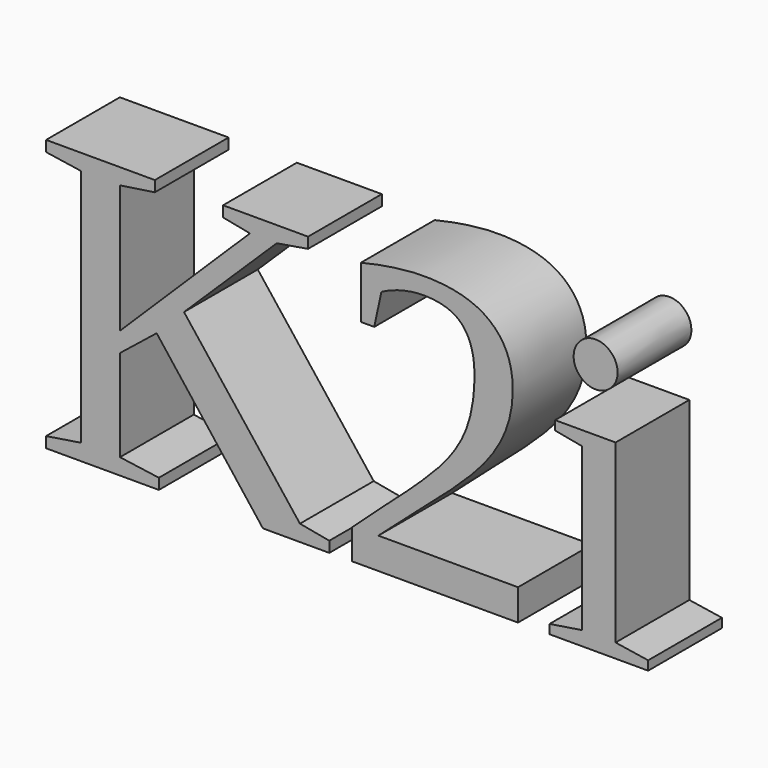
from build123d import *

# Parameters (mm, degrees)
F0_TEXT_SIZE = 44.9661579397
F1_DEPTH     = 10


# Not quite as in the source:
# - Text() gives the source's letters only with a copy of the font that has no kerning and outlines rounded to 1/6400 em; it was checked with that copy


with BuildPart() as f1:
    # F0 (on Front) → F1 (new body)
    with BuildSketch(Plane.XZ):
        with Locations((0, 0)):
            Text('K2i', F0_TEXT_SIZE, font='Tinos', text_align=(TextAlign.LEFT, TextAlign.BOTTOM))
    extrude(amount=F1_DEPTH)


solid = f1.part
